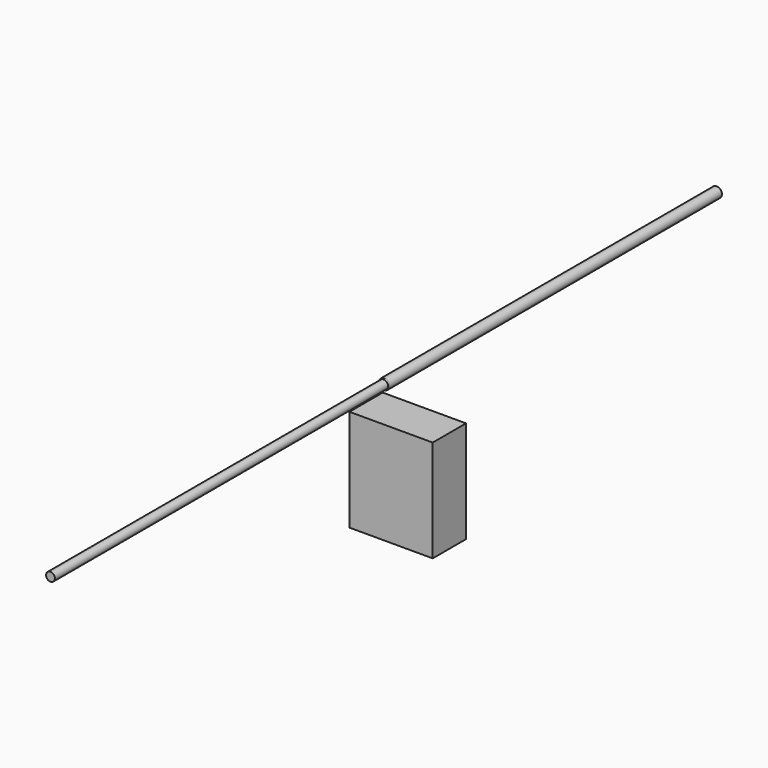
from build123d import *

# Parameters (mm, degrees)
F0_R     = 32.0315478489
F1_DEPTH = 2540
F2_R     = 5.08
F3_DEPTH = 2541.625266
F4_W     = 508
F4_H     = 254
F5_DEPTH = 622.3


# Not quite as in the source:
# - an extrude ends at something that could not be found from the text; its depth is read off the source's solid


with BuildPart() as f1:
    # F0 (on Front) → F1 (new body)
    with BuildSketch(Plane.XZ):
        Circle(F0_R)
    extrude(amount=F1_DEPTH)

    # F2
    f2_edges = [f1.edges().sort_by_distance(p)[0] for p in [
        (-32.031548, -2540, 0),
    ]]
    fillet(f2_edges, radius=F2_R)

    # F3 (add, through all): a face of the model
    f3_faces = [f1.faces().sort_by_distance(p)[0] for p in [
        (0, -2540, 0),
    ]]
    extrude(f3_faces, amount=F3_DEPTH)


with BuildPart() as f5:
    # F4 (on Top) → F5 (new body)
    with BuildSketch(Plane.XY):
        with Locations((303.0977845192, -2735.4523357783)):
            Rectangle(F4_W, F4_H)
    extrude(amount=-F5_DEPTH)


solid = Compound([f1.part, f5.part])
